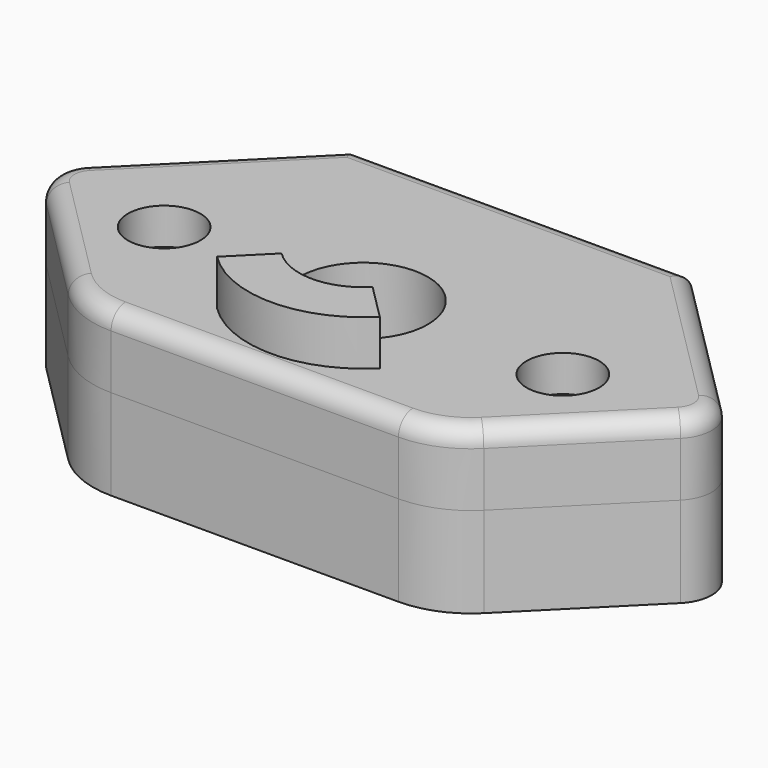
from build123d import *

# Parameters (mm, degrees)
F0_W            = 20
F0_H            = 15
F1_DEPTH        = 5
F2_R            = 1
F2_W            = 13
F2_H            = 12
F3_DEPTH        = 5
F4_W            = 6
F4_H            = 12
F5_DEPTH        = 0.5
F7_DEPTH        = 4
F8_R            = 3.55
F9_DEPTH        = 4
F10_R           = 1
F11_D           = 2
F11_DEPTH       = 20
F11_CBORE_D     = 4
F11_CBORE_DEPTH = 2
F11_TIP         = 0.600860619
F12_F1_R        = 5
F12_F2_R        = 5
F12_2_T1_DEPTH  = 9.1776695297
F12_2_T4_ANGLE  = 45
F12_2_T6_ANGLE  = 45
F13_R           = 2
F15_T1_DEPTH    = 9
F15_T4_ANGLE    = 90
F15_T6_ANGLE    = 90
F17_DEPTH       = 2.5


# Not quite as in the source:
# - a fillet or chamfer that OpenCascade refuses, or shapes differently, is made with other operations: its cross-section is extruded or revolved along the edge and cut away or added
# - two fillets or chamfers of one size are made in one step


with BuildPart() as f1:
    # F0 (on Top) → F1 (new body)
    with BuildSketch(Plane.XY):
        with Locations((0, 7.5)):
            Rectangle(F0_W, F0_H)
        Polygon((17.5, 7.5), (10, 15), (10, 0), align=None)
        Polygon((6.5, 18.5), (10, 15), (17.5, 7.5), (18.9142135624, 8.9142135624), (9.3284271247, 18.5), align=None)
        Polygon((-10, 15), (10, 15), (6.5, 18.5), (-6.5, 18.5), align=None)
        Polygon((-10, 0), (-10, 15), (-17.5, 7.5), align=None)
        Polygon((-17.5, 7.5), (-10, 15), (-6.5, 18.5), (-9.3284271247, 18.5), (-18.9142135624, 8.9142135624), align=None)
    extrude(amount=F1_DEPTH)

    # F2 (on face) → F3 (cut)
    with BuildSketch(Plane.XY.offset(5)):
        with Locations((-11, 7.5)):
            Circle(F2_R)
        with Locations((11, 7.5)):
            Circle(F2_R)
        with Locations((0, 7.5)):
            Rectangle(F2_W, F2_H)
    extrude(amount=-F3_DEPTH, mode=Mode.SUBTRACT)

    # F4 (on face) → F5 (join)
    with BuildSketch(Plane(origin=(0, 0, 0), x_dir=(1, 0, 0), z_dir=(0, 0, -1))):
        with Locations((0, -7.5)):
            Rectangle(F4_W, F4_H)
    extrude(amount=-F5_DEPTH)

    # F12: fillet of radius 5 on 2 edges, made by hand

    # F12_f1
    f12_f1_edges = [f1.edges().sort_by_distance(p)[0] for p in [
        (-10, 0, 2.5),
    ]]
    fillet(f12_f1_edges, radius=F12_F1_R)

    # F12_f2
    f12_f2_edges = [f1.edges().sort_by_distance(p)[0] for p in [
        (10, 0, 2.5),
    ]]
    fillet(f12_f2_edges, radius=F12_F2_R)

    # F13
    f13_edges = [f1.edges().sort_by_distance(p)[0] for p in [
        (-18.914214, 8.914214, 2.5),
        (18.914214, 8.914214, 2.5),
    ]]
    fillet(f13_edges, radius=F13_R)


with BuildPart() as f7:
    # F6 (on face) → F7 (new body)
    with BuildSketch(Plane.XY.offset(5)):
        Polygon((-18.9142135624, 8.9142135624), (-10, 0), (10, 0), (18.9142135624, 8.9142135624), (9.3284271247, 18.5), (-9.3284271247, 18.5), align=None)
    extrude(amount=F7_DEPTH)

    # F8 (on face) → F9 (cut)
    with BuildSketch(Plane.XY.offset(9)):
        with Locations((0, 7.5)):
            Circle(F8_R)
    extrude(amount=-F9_DEPTH, mode=Mode.SUBTRACT)

    # F10
    f10_edges = [f7.edges().sort_by_distance(p)[0] for p in [
        (-14.457107, 4.457107, 9),
        (0, 0, 9),
        (14.457107, 4.457107, 9),
        (14.12132, 13.707107, 9),
        (0, 18.5, 9),
        (-14.12132, 13.707107, 9),
    ]]
    fillet(f10_edges, radius=F10_R)

    # F11
    with Locations(Plane.XY.offset(9)):
        with Locations((11, 7.5), (-11, 7.5)):
            CounterBoreHole(F11_D / 2, F11_CBORE_D / 2, F11_CBORE_DEPTH, depth=F11_DEPTH)
            with Locations((0, 0, -(F11_DEPTH + F11_TIP / 2))):  # 118° drill point
                Cone(0, F11_D / 2, F11_TIP, mode=Mode.SUBTRACT)

    # F12#2: fillet of radius 5 on 2 edges, made by hand

    # F12_2_s2 → F12_2_t1 (cut)
    with BuildSketch(Plane.XY.offset(-0.1776695297)):
        with BuildLine():
            ThreePointArc((-11.4644660941, 1.4644660941), (-9.84234935, 0.3806023374), (-7.9289321881, 0))
            Line((-7.9289321881, 0), (-10, 0))
            Line((-10, 0), (-11.4644660941, 1.4644660941))
        make_face()
        with BuildLine():
            ThreePointArc((7.9289321881, 0), (9.84234935, 0.3806023374), (11.4644660941, 1.4644660941))
            Line((11.4644660941, 1.4644660941), (10, 0))
            Line((10, 0), (7.9289321881, 0))
        make_face()
    extrude(amount=F12_2_T1_DEPTH, mode=Mode.SUBTRACT)

    # F12_2_s3 → F12_2_t4 (revolve, cut)
    with BuildSketch(Plane.YZ.offset(7.9289321881)):
        with BuildLine():
            ThreePointArc((1, 9), (0.2928932188, 8.7071067812), (0, 8))
            Line((0, 8), (0, 9))
            Line((0, 9), (1, 9))
        make_face()
    revolve(axis=Axis((7.9289321881, 5, 9), (0, 0, 1)), revolution_arc=F12_2_T4_ANGLE, mode=Mode.SUBTRACT)

    # F12_2_s5 → F12_2_t6 (revolve, cut)
    with BuildSketch(Plane(origin=(-6.4644660941, 6.4644660941, 0), x_dir=(0, 0, 1), z_dir=(-0.7071067812, 0.7071067812, 0))):
        with BuildLine():
            ThreePointArc((9, -6.0710678119), (8.7071067812, -6.7781745931), (8, -7.0710678119))
            Line((8, -7.0710678119), (9, -7.0710678119))
            Line((9, -7.0710678119), (9, -6.0710678119))
        make_face()
    revolve(axis=Axis((-7.9289321881, 5, 9), (0, 0, 1)), revolution_arc=F12_2_T6_ANGLE, mode=Mode.SUBTRACT)

    # F15: fillet of radius 2 on 2 edges, made by hand

    # F15_s2 → F15_t1 (cut)
    with BuildSketch(Plane.XY):
        with BuildLine():
            ThreePointArc((-17.5, 7.5), (-18.0857864376, 8.9142135624), (-17.5, 10.3284271247))
            Line((-17.5, 10.3284271247), (-18.9142135624, 8.9142135624))
            Line((-18.9142135624, 8.9142135624), (-17.5, 7.5))
        make_face()
        with BuildLine():
            ThreePointArc((17.5, 10.3284271247), (18.0857864376, 8.9142135624), (17.5, 7.5))
            Line((17.5, 7.5), (18.9142135624, 8.9142135624))
            Line((18.9142135624, 8.9142135624), (17.5, 10.3284271247))
        make_face()
    extrude(amount=F15_T1_DEPTH, mode=Mode.SUBTRACT)

    # F15_s3 → F15_t4 (revolve, cut)
    with BuildSketch(Plane(origin=(12.5, 12.5, 0), x_dir=(0, 0, 1), z_dir=(-0.7071067812, -0.7071067812, 0))):
        with BuildLine():
            ThreePointArc((9, -6.0710678119), (8.7071067812, -6.7781745931), (8, -7.0710678119))
            Line((8, -7.0710678119), (9, -7.0710678119))
            Line((9, -7.0710678119), (9, -6.0710678119))
        make_face()
    revolve(axis=Axis((16.0857864376, 8.9142135624, 9), (0, 0, 1)), revolution_arc=F15_T4_ANGLE, mode=Mode.SUBTRACT)

    # F15_s5 → F15_t6 (revolve, cut)
    with BuildSketch(Plane(origin=(-3.5857864376, -3.5857864376, 0), x_dir=(0, 0, 1), z_dir=(0.7071067812, 0.7071067812, 0))):
        with BuildLine():
            ThreePointArc((9, -18.6776695297), (8.7071067812, -19.3847763109), (8, -19.6776695297))
            Line((8, -19.6776695297), (9, -19.6776695297))
            Line((9, -19.6776695297), (9, -18.6776695297))
        make_face()
    revolve(axis=Axis((-16.0857864376, 8.9142135624, 9), (0, 0, 1)), revolution_arc=F15_T6_ANGLE, mode=Mode.SUBTRACT)

    # F16 (on face) → F17 (join)
    with BuildSketch(Plane.XY.offset(9)):
        with BuildLine():
            Line((-2.5102290732, 4.9897709268), (-4.4901280605, 3.0098719395))
            ThreePointArc((-4.4901280605, 3.0098719395), (0, 1.15), (4.4901280605, 3.0098719395))
            Line((4.4901280605, 3.0098719395), (2.5102290732, 4.9897709268))
            ThreePointArc((2.5102290732, 4.9897709268), (0, 3.95), (-2.5102290732, 4.9897709268))
        make_face()
    extrude(amount=F17_DEPTH)


solid = Compound([f1.part, f7.part])
